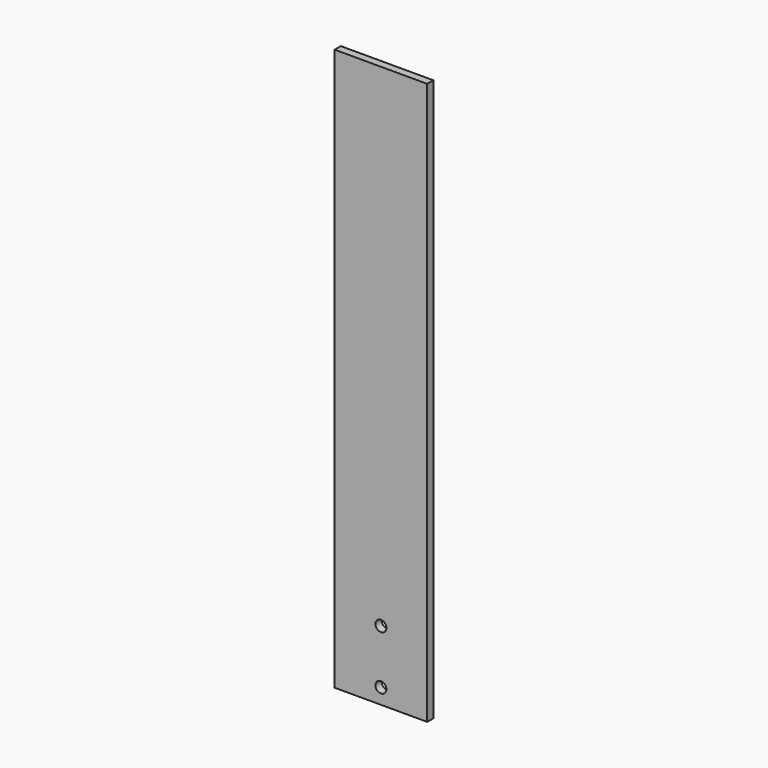
from build123d import *

# Parameters (mm, degrees)
F0_W     = 38.1
F0_H     = 231.14
F1_DEPTH = 3.175
F3_D     = 4.4958


# Not quite as in the source:
# - a length typed as a fraction of an inch, garbled in the dataset ("3 / 203.2 mm" for 3/8 in), is restored


with BuildPart() as f1:
    # F0 (on Front) → F1 (new body)
    with BuildSketch(Plane.XZ):
        with Locations((-19.05, 115.57)):
            Rectangle(F0_W, F0_H)
    extrude(amount=F1_DEPTH)

    # F3 (through all)
    with Locations(Plane(origin=(0, 0, 0), x_dir=(-1, 0, 0), z_dir=(0, 1, 0))):
        with Locations((19.05, 6.35), (19.05, 28.575)):
            Hole(F3_D / 2)


solid = f1.part
